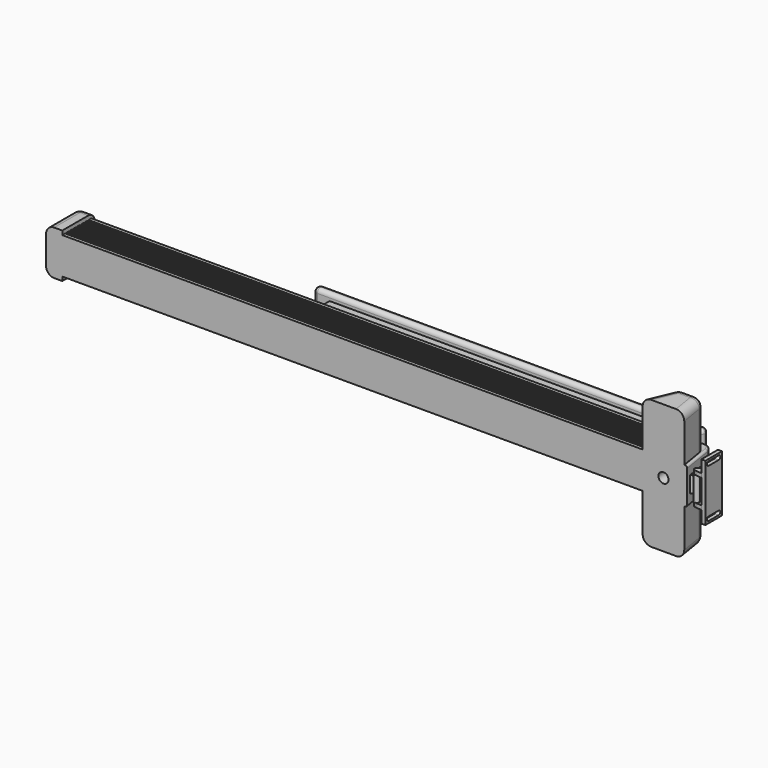
from build123d import *

# Parameters (mm, degrees)
F0_W           = 911.225
F0_H           = 57.15
F1_DEPTH       = 57.15
F3_DEPTH       = 57.15
F5_R           = 3.175
F6_DEPTH       = 130.175
F6_DEPTH_BACK  = 73.025
F7_R           = 12.7
F9_DEPTH       = 911.225
F10_W          = 63.5
F10_H          = 69.85
F11_DEPTH      = 25.4
F12_R          = 12.7
F13_R          = 12.7
F14_W          = 558.8
F14_H          = 35.71875
F15_DEPTH      = 25.4
F15_DEPTH_BACK = 26.9875
F16_W          = 609.6
F16_H          = 57.15
F17_DEPTH      = 12.7
F18_R          = 6.34999
F19_R          = 7.9375
F20_DEPTH      = 25.4
F24_DEPTH      = 12.7
F24_DEPTH_BACK = 12.7
F26_DEPTH      = 25.4
F26_DEPTH_BACK = 25.4
F29_DEPTH      = 6.35
F30_DEPTH      = 6.35
F31_DEPTH      = 19.05
F31_DEPTH_BACK = 19.05
F32_DEPTH      = 44.45
F32_DEPTH_BACK = 44.45
F34_DEPTH      = 6.2889696488


# Not quite as in the source:
# - a fillet or chamfer is up to 0.001 mm smaller than in the source, because OpenCascade refuses the exact size


with BuildPart() as f1:
    # F0 (on Front) → F1 (new body)
    with BuildSketch(Plane.XZ):
        with Locations((-455.6125, 28.575)):
            Rectangle(F0_W, F0_H)
    extrude(amount=-F1_DEPTH)

    # F2 (on Top) → F3 (join, through all)
    with BuildSketch(Plane.XY):
        with BuildLine():
            Line((0, 60.325), (0, 0))
            Line((0, 0), (69.85, 0))
            Line((69.85, 0), (61.7171543383, 49.6768641398))
            ThreePointArc((61.7171543383, 49.6768641398), (57.4068785119, 57.3035503712), (49.1840041536, 60.325))
            Line((49.1840041536, 60.325), (0, 60.325))
        make_face()
    extrude(amount=F3_DEPTH)

    # F5
    f5_edges = [f1.edges().sort_by_distance(p)[0] for p in [
        (24.592002, 60.325, 0),
        (24.592002, 60.325, 57.15),
    ]]
    fillet(f5_edges, radius=F5_R)

    # F4 (on Top) → F6 (join, two sides)
    with BuildSketch(Plane.XY) as f6_sk:
        with BuildLine():
            Line((0, 0), (65.2439892292, 0))
            Line((65.2439892292, 0), (59.260224713, 36.5498952375))
            ThreePointArc((59.260224713, 36.5498952375), (54.9499488866, 44.1765814688), (46.7270745283, 47.1980310977))
            Line((46.7270745283, 47.1980310977), (28.5304468125, 47.1980310977))
            ThreePointArc((28.5304468125, 47.1980310977), (21.5310864577, 45.0951512075), (16.8496495885, 39.4829058414))
            Line((16.8496495885, 39.4829058414), (0, 0))
        make_face()
    extrude(amount=F6_DEPTH)
    extrude(f6_sk.sketch, amount=-F6_DEPTH_BACK)

    # F7
    f7_edges = [f1.edges().sort_by_distance(p)[0] for p in [
        (8.424825, 19.741453, 130.175),
        (8.424825, 19.741453, -73.025),
    ]]
    fillet(f7_edges, radius=F7_R)

    # F8 (on face) → F9 (cut, through all)
    with BuildSketch(Plane(origin=(-911.225, 0, 0), x_dir=(0, -1, 0), z_dir=(-1, 0, 0))):
        with BuildLine():
            Line((-51.59375, 0), (-48.41875, 0))
            ThreePointArc((-48.41875, 0), (-50.00625, 1.5875), (-51.59375, 0))
        make_face()
        with BuildLine():
            Line((-44.45, 0), (-41.275, 0))
            ThreePointArc((-41.275, 0), (-42.8625, 1.5875), (-44.45, 0))
        make_face()
        with BuildLine():
            Line((-37.30625, 0), (-34.13125, 0))
            ThreePointArc((-34.13125, 0), (-35.71875, 1.5875), (-37.30625, 0))
        make_face()
        with BuildLine():
            Line((-30.1625, 0), (-26.9875, 0))
            ThreePointArc((-26.9875, 0), (-28.575, 1.5875), (-30.1625, 0))
        make_face()
        with BuildLine():
            Line((-23.01875, 0), (-19.84375, 0))
            ThreePointArc((-19.84375, 0), (-21.43125, 1.5875), (-23.01875, 0))
        make_face()
        with BuildLine():
            Line((-15.875, 0), (-12.7, 0))
            ThreePointArc((-12.7, 0), (-14.2875, 1.5875), (-15.875, 0))
        make_face()
        with BuildLine():
            Line((-8.73125, 0), (-5.55625, 0))
            ThreePointArc((-5.55625, 0), (-7.14375, 1.5875), (-8.73125, 0))
        make_face()
        with BuildLine():
            Line((-57.15, 8.73125), (-57.15, 5.55625))
            ThreePointArc((-57.15, 5.55625), (-55.5625, 7.14375), (-57.15, 8.73125))
        make_face()
        with BuildLine():
            ThreePointArc((-51.59375, 57.15), (-50.00625, 55.5625), (-48.41875, 57.15))
            Line((-48.41875, 57.15), (-51.59375, 57.15))
        make_face()
        with BuildLine():
            ThreePointArc((-37.30625, 57.15), (-35.71875, 55.5625), (-34.13125, 57.15))
            Line((-34.13125, 57.15), (-37.30625, 57.15))
        make_face()
        with BuildLine():
            ThreePointArc((-44.45, 57.15), (-42.8625, 55.5625), (-41.275, 57.15))
            Line((-41.275, 57.15), (-44.45, 57.15))
        make_face()
        with BuildLine():
            ThreePointArc((-30.1625, 57.15), (-28.575, 55.5625), (-26.9875, 57.15))
            Line((-26.9875, 57.15), (-30.1625, 57.15))
        make_face()
        with BuildLine():
            ThreePointArc((-8.73125, 57.15), (-7.14375, 55.5625), (-5.55625, 57.15))
            Line((-5.55625, 57.15), (-8.73125, 57.15))
        make_face()
        with BuildLine():
            ThreePointArc((-23.01875, 57.15), (-21.43125, 55.5625), (-19.84375, 57.15))
            Line((-19.84375, 57.15), (-23.01875, 57.15))
        make_face()
        with BuildLine():
            ThreePointArc((-15.875, 57.15), (-14.2875, 55.5625), (-12.7, 57.15))
            Line((-12.7, 57.15), (-15.875, 57.15))
        make_face()
        with BuildLine():
            Line((-57.15, 15.875), (-57.15, 12.7))
            ThreePointArc((-57.15, 12.7), (-55.5625, 14.2875), (-57.15, 15.875))
        make_face()
        with BuildLine():
            Line((-57.15, 23.01875), (-57.15, 19.84375))
            ThreePointArc((-57.15, 19.84375), (-55.5625, 21.43125), (-57.15, 23.01875))
        make_face()
        with BuildLine():
            Line((-57.15, 30.1625), (-57.15, 26.9875))
            ThreePointArc((-57.15, 26.9875), (-55.5625, 28.575), (-57.15, 30.1625))
        make_face()
        with BuildLine():
            Line((-57.15, 37.30625), (-57.15, 34.13125))
            ThreePointArc((-57.15, 34.13125), (-55.5625, 35.71875), (-57.15, 37.30625))
        make_face()
        with BuildLine():
            Line((-57.15, 44.45), (-57.15, 41.275))
            ThreePointArc((-57.15, 41.275), (-55.5625, 42.8625), (-57.15, 44.45))
        make_face()
        with BuildLine():
            Line((-57.15, 51.59375), (-57.15, 48.41875))
            ThreePointArc((-57.15, 48.41875), (-55.5625, 50.00625), (-57.15, 51.59375))
        make_face()
    extrude(amount=-F9_DEPTH, mode=Mode.SUBTRACT)

    # F10 (on face) → F11 (join)
    with BuildSketch(Plane(origin=(-911.225, 0, 0), x_dir=(0, -1, 0), z_dir=(-1, 0, 0))):
        with Locations((-31.75, 28.575)):
            Rectangle(F10_W, F10_H)
    extrude(amount=F11_DEPTH)

    # F12
    f12_edges = [f1.edges().sort_by_distance(p)[0] for p in [
        (-923.925, 63.5, -6.35),
        (-923.925, 63.5, 63.5),
    ]]
    fillet(f12_edges, radius=F12_R)

    # F13
    f13_edges = [f1.edges().sort_by_distance(p)[0] for p in [
        (-936.625, 25.4, 63.5),
    ]]
    fillet(f13_edges, radius=F13_R)

    # F14 (on face) → F15 (join, two sides)
    with BuildSketch(Plane(origin=(0, 57.15, 0), x_dir=(-1, 0, 0), z_dir=(0, 1, 0))) as f15_sk:
        with Locations((279.4, 28.575)):
            Rectangle(F14_W, F14_H)
    extrude(amount=-F15_DEPTH)
    extrude(f15_sk.sketch, amount=F15_DEPTH_BACK)

    # F16 (on face) → F17 (join)
    with BuildSketch(Plane(origin=(0, 84.1375, 0), x_dir=(-1, 0, 0), z_dir=(0, 1, 0))):
        with Locations((279.4, 28.575)):
            Rectangle(F16_W, F16_H)
    extrude(amount=F17_DEPTH)

    # F18 (radius 6.35 in the source; OpenCascade refuses exactly that, so slightly less here)
    f18_edges = [f1.edges().sort_by_distance(p)[0] for p in [
        (-279.4, 96.8375, 57.15),
        (25.4, 96.8375, 28.575),
        (-279.4, 96.8375, 0),
        (-279.4, 84.1375, 0),
        (25.4, 84.1375, 28.575),
        (25.4, 90.4875, 0),
        (25.4, 90.4875, 57.15),
        (-584.2, 84.1375, 28.575),
        (-584.2, 96.8375, 28.575),
        (-584.2, 90.4875, 0),
        (-584.2, 90.4875, 57.15),
        (-279.4, 84.1375, 57.15),
    ]]
    fillet(f18_edges, radius=F18_R)

    # F19 (on face) → F20 (cut)
    with BuildSketch(Plane.XZ):
        with Locations((32.6219946146, 28.575)):
            Circle(F19_R)
    extrude(amount=-F20_DEPTH, mode=Mode.SUBTRACT)

    # F23 (on plane+point) → F24 (join, two sides)
    with BuildSketch(Plane.XY.offset(28.5750000002)) as f24_sk:
        with BuildLine():
            Line((84.6916779676, 18.4073803931), (63.6300831519, 37.9923555759))
            Line((63.6300831519, 37.9923555759), (68.646088853, 7.3537028705))
            ThreePointArc((68.646088853, 7.3537028705), (77.275044264, 12.0006346528), (84.6916779676, 18.4073803931))
        make_face()
    extrude(amount=F24_DEPTH)
    extrude(f24_sk.sketch, amount=-F24_DEPTH_BACK)


with BuildPart() as f26:
    # F25 (on plane+point) → F26 (new body, two sides)
    with BuildSketch(Plane.XY.offset(28.5750000002)) as f26_sk:
        Polygon((91.3757458329, 33.3596840501), (91.3757458329, 28.8400221616), (91.3757458329, 0.8469638929), (97.6637154818, 0.8469638929), (97.6637154818, 33.3596840501), align=None)
    extrude(amount=F26_DEPTH)
    extrude(f26_sk.sketch, amount=-F26_DEPTH_BACK)

    # F27 (on face) → F29 (join)
    with BuildSketch(Plane(origin=(0, 0, 3.1750000002), x_dir=(1, 0, 0), z_dir=(0, 0, -1))):
        with BuildLine():
            ThreePointArc((91.3757458329, -0.8469638929), (86.7120292767, -1.0590698667), (82.0868194172, -1.6936365026))
            ThreePointArc((82.0868194172, -1.6936365026), (84.4594186062, -6.113912923), (80.8473515261, -9.5954416035))
            ThreePointArc((80.8473515261, -9.5954416035), (88.5716049262, -17.8718754684), (91.3757458329, -28.8400221616))
            Line((91.3757458329, -28.8400221616), (91.3757458329, -0.8469638929))
        make_face()
        with BuildLine():
            ThreePointArc((80.8473515261, -9.5954416035), (84.4594186062, -6.113912923), (82.0868194172, -1.6936365026))
            ThreePointArc((82.0868194172, -1.6936365026), (80.8342972281, -1.9400043566), (79.5882823189, -2.2174134402))
            ThreePointArc((79.5882823189, -2.2174134402), (77.036630058, -5.0747288341), (78.8455087226, -8.4515821767))
            ThreePointArc((78.8455087226, -8.4515821767), (79.8608648567, -8.9982499879), (80.8473515261, -9.5954416035))
        make_face()
    extrude(amount=-F29_DEPTH)

    # F28 (on face) → F30 (join)
    with BuildSketch(Plane.XY.offset(53.9750000002)):
        with BuildLine():
            ThreePointArc((80.8473515261, 9.5954416035), (84.4594186062, 6.113912923), (82.0868194172, 1.6936365026))
            ThreePointArc((82.0868194172, 1.6936365026), (86.7120292767, 1.0590698667), (91.3757458329, 0.8469638929))
            Line((91.3757458329, 0.8469638929), (91.3757458329, 28.8400221616))
            ThreePointArc((91.3757458329, 28.8400221616), (88.5716049262, 17.8718754684), (80.8473515261, 9.5954416035))
        make_face()
        with BuildLine():
            ThreePointArc((79.5882823189, 2.2174134402), (80.8342972281, 1.9400043566), (82.0868194172, 1.6936365026))
            ThreePointArc((82.0868194172, 1.6936365026), (84.4594186062, 6.113912923), (80.8473515261, 9.5954416035))
            ThreePointArc((80.8473515261, 9.5954416035), (79.8608648567, 8.9982499879), (78.8455087226, 8.4515821767))
            ThreePointArc((78.8455087226, 8.4515821767), (77.036630058, 5.0747288341), (79.5882823189, 2.2174134402))
        make_face()
    extrude(amount=-F30_DEPTH)

    # F25 (on plane+point) → F31 (join, two sides)
    with BuildSketch(Plane.XY.offset(28.5750000002)) as f31_sk:
        with BuildLine():
            ThreePointArc((78.8455087226, 8.4515821767), (79.8608648567, 8.9982499879), (80.8473515261, 9.5954416035))
            ThreePointArc((80.8473515261, 9.5954416035), (76.2505436426, 4.826278413), (82.0868194172, 1.6936365026))
            ThreePointArc((82.0868194172, 1.6936365026), (80.8342972281, 1.9400043566), (79.5882823189, 2.2174134402))
            ThreePointArc((79.5882823189, 2.2174134402), (77.036630058, 5.0747288341), (78.8455087226, 8.4515821767))
        make_face()
        with BuildLine():
            ThreePointArc((82.0868194172, 1.6936365026), (83.8518401521, 3.2266865121), (84.5096059811, 5.470095668))
            ThreePointArc((84.5096059811, 5.470095668), (83.4619508708, 8.2282919437), (80.8473515261, 9.5954416035))
            ThreePointArc((80.8473515261, 9.5954416035), (79.8608648567, 8.9982499879), (78.8455087226, 8.4515821767))
            ThreePointArc((78.8455087226, 8.4515821767), (77.036630058, 5.0747288341), (79.5882823189, 2.2174134402))
            ThreePointArc((79.5882823189, 2.2174134402), (80.8342972281, 1.9400043566), (82.0868194172, 1.6936365026))
        make_face()
    extrude(amount=F31_DEPTH)
    extrude(f31_sk.sketch, amount=-F31_DEPTH_BACK)

    # F25 (on plane+point) → F32 (join, two sides)
    with BuildSketch(Plane.XY.offset(28.5750000002)) as f32_sk:
        Polygon((91.3757458329, 33.3596840501), (91.3757458329, 28.8400221616), (91.3757458329, 0.8469638929), (97.6637154818, 0.8469638929), (97.6637154818, 33.3596840501), align=None)
    extrude(amount=F32_DEPTH)
    extrude(f32_sk.sketch, amount=-F32_DEPTH_BACK)

    # F33 (on face) → F34 (cut, through all)
    with BuildSketch(Plane(origin=(91.3757458329, 0, 0), x_dir=(0, -1, 0), z_dir=(-1, 0, 0))):
        with BuildLine():
            Line((-27.0096840501, -12.6999999998), (-7.1969638929, -12.6999999998))
            ThreePointArc((-7.1969638929, -12.6999999998), (-4.0219638929, -9.5249999998), (-7.1969638929, -6.3499999998))
            Line((-7.1969638929, -6.3499999998), (-27.0096840501, -6.3499999998))
            ThreePointArc((-27.0096840501, -6.3499999998), (-30.1846840501, -9.5249999998), (-27.0096840501, -12.6999999998))
        make_face()
        with BuildLine():
            Line((-27.0096840501, 63.5000000002), (-7.1969638929, 63.5000000002))
            ThreePointArc((-7.1969638929, 63.5000000002), (-4.0219638929, 66.6750000002), (-7.1969638929, 69.8500000002))
            Line((-7.1969638929, 69.8500000002), (-27.0096840501, 69.8500000002))
            ThreePointArc((-27.0096840501, 69.8500000002), (-30.1846840501, 66.6750000002), (-27.0096840501, 63.5000000002))
        make_face()
    extrude(amount=-F34_DEPTH, mode=Mode.SUBTRACT)


solid = Compound([f1.part, f26.part])
